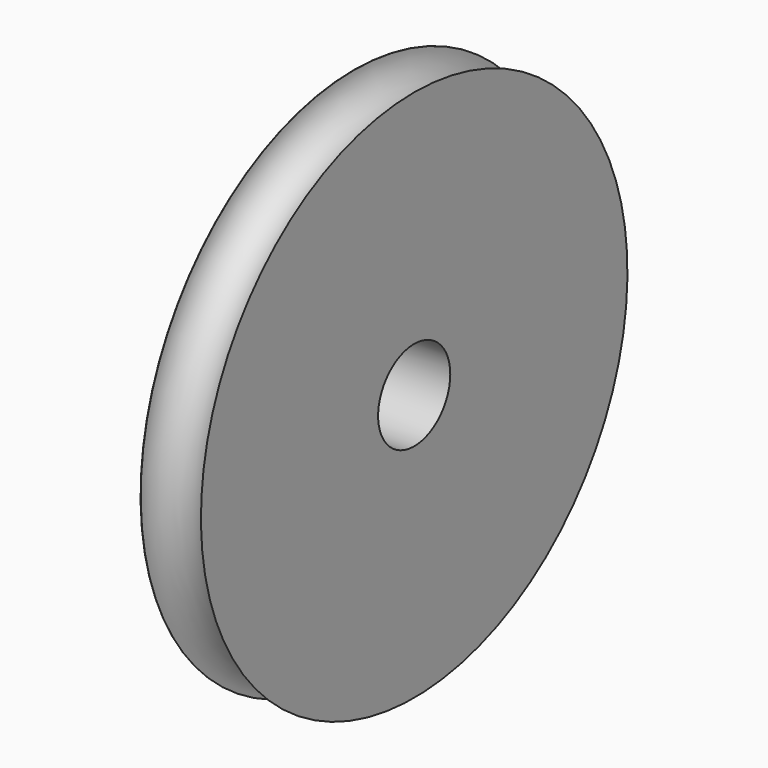
from build123d import *

# Parameters (mm, degrees)
F2_R     = 1.5875
F3_DEPTH = 3.175


# Not quite as in the source:
# - a length typed as a fraction of an inch, garbled in the dataset ("3 / 203.2 mm" for 3/8 in), is restored


with BuildPart() as f1:
    # F0 (on Front) → F1 (revolve)
    with BuildSketch(Plane.XZ):
        with BuildLine():
            Line((1.059713671, 0), (1.059713671, 9.3838354061))
            ThreePointArc((1.059713671, 9.3838354061), (1e-10, 8.3241217351), (-1.059713671, 9.3838354058))
            ThreePointArc((-1.0597136683, 9.3838354055), (-1.0630601457, 9.3834601649), (-1.0664064903, 9.3830837412))
            Line((-1.0664064903, 9.3830837412), (-1.0664064903, 0))
            Line((-1.0664064903, 0), (1.059713671, 0))
        make_face()
    revolve(axis=Axis((-0.0033464096, 0, 0), (1, 0, 0)))

    # F2 (on Right) → F3 (cut, symmetric)
    with BuildSketch(Plane.YZ):
        Circle(F2_R)
    extrude(amount=F3_DEPTH, both=True, mode=Mode.SUBTRACT)


solid = f1.part
